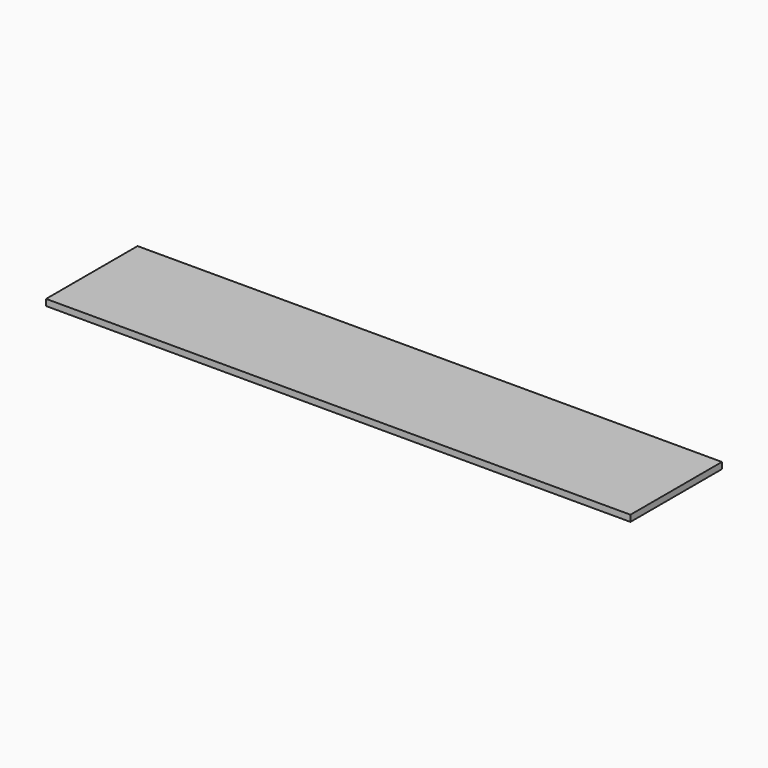
from build123d import *

# Parameters (mm, degrees)
F0_W     = 292.1
F0_H     = 57.15
F1_DEPTH = 3.175


# Not quite as in the source:
# - a length typed as a fraction of an inch, garbled in the dataset ("3 / 203.2 mm" for 3/8 in), is restored


with BuildPart() as f1:
    # F0 (on Top) → F1 (new body)
    with BuildSketch(Plane.XY):
        Rectangle(F0_W, F0_H)
    extrude(amount=F1_DEPTH)


solid = f1.part
